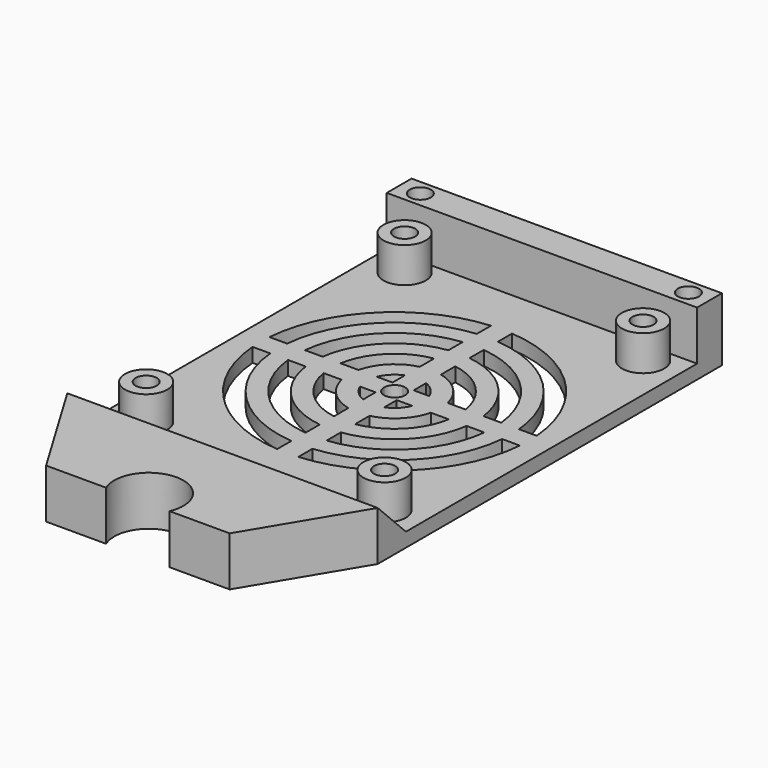
from build123d import *

# Parameters (mm, degrees)
F0_W        = 44
F0_H        = 61
F1_DEPTH    = 2
F3_DEPTH    = 7
F4_R        = 3
F4_R_2      = 1.5
F5_DEPTH    = 5
F6_T4_DEPTH = 44
F7_W        = 44
F7_H        = 4.4
F8_DEPTH    = 7
F9_R        = 1.5
F10_DEPTH   = 7
F12_DEPTH   = 2.001


# Not quite as in the source:
# - a fillet or chamfer that OpenCascade refuses, or shapes differently, is made with other operations: its cross-section is extruded or revolved along the edge and cut away or added


with BuildPart() as f1:
    # F0 (on Top) → F1 (new body)
    with BuildSketch(Plane.XY):
        Rectangle(F0_W, F0_H)
    extrude(amount=F1_DEPTH)

    # F2 (on face) → F3 (join)
    with BuildSketch(Plane(origin=(0, 0, 0), x_dir=(1, 0, 0), z_dir=(0, 0, -1))):
        with BuildLine():
            Line((-13.0117940697, 45.5), (-22, 30.5))
            Line((-22, 30.5), (22, 30.5))
            Line((22, 30.5), (13.0117940697, 45.5))
            Line((13.0117940697, 45.5), (4.5, 45.5))
            ThreePointArc((4.5, 45.5), (0, 38.660928057), (-4.5, 45.5))
            Line((-4.5, 45.5), (-13.0117940697, 45.5))
        make_face()
    extrude(amount=-F3_DEPTH)

    # F4 (on face) → F5 (join)
    with BuildSketch(Plane.XY.offset(2)):
        with Locations((-16.9, 22.9)):
            Circle(F4_R)
        with Locations((-16.9, 22.9)):
            Circle(F4_R_2, mode=Mode.SUBTRACT)
        with Locations((16.9, 22.9)):
            Circle(F4_R)
        with Locations((16.9, 22.9)):
            Circle(F4_R_2, mode=Mode.SUBTRACT)
        with Locations((16.9, -22.9)):
            Circle(F4_R)
        with Locations((16.9, -22.9)):
            Circle(F4_R_2, mode=Mode.SUBTRACT)
        with Locations((-16.9, -22.9)):
            Circle(F4_R)
        with Locations((-16.9, -22.9)):
            Circle(F4_R_2, mode=Mode.SUBTRACT)
    extrude(amount=F5_DEPTH)

    # F6: chamfer of 5 on 1 edges, made by hand


with BuildPart() as f6_tool2:
    # F6_s3 → F6_t4 (new body)
    with BuildSketch(Plane.YZ.offset(-22)):
        Polygon((-25.5, 2), (-30.5, 7), (-30.5, 2), align=None)
    extrude(amount=F6_T4_DEPTH)

    split(bisect_by=Plane(origin=(29.6352662025, -17.7578583619, 0), x_dir=(0, 0, 1), z_dir=(-0.8577903364, 0.5139997459, 0)), keep=Keep.TOP)

    split(bisect_by=Plane.XY.offset(7), keep=Keep.BOTTOM)

    split(bisect_by=Plane(origin=(-29.6352662025, -17.7578583619, 0), x_dir=(0, 0, 1), z_dir=(0.8577903364, 0.5139997459, 0)), keep=Keep.TOP)


with BuildPart() as f1_1:
    add(f1.part)

    # F6_t1: union F6_tool2
    add(f6_tool2.part)

    # F7 (on face) → F8 (join)
    with BuildSketch(Plane.XY.offset(2)):
        with Locations((0, 28.3)):
            Rectangle(F7_W, F7_H)
    extrude(amount=F8_DEPTH)

    # F9 (on face) → F10 (cut)
    with BuildSketch(Plane.XY.offset(9)):
        with Locations((-19, 28.3)):
            Circle(F9_R)
        with Locations((19, 28.3)):
            Circle(F9_R)
    extrude(amount=-F10_DEPTH, mode=Mode.SUBTRACT)

    # F11 (on face) → F12 (cut, through all)
    with BuildSketch(Plane.XY.offset(2)):
        with BuildLine():
            Line((16.4316767252, 1.5), (18.9406969249, 1.5))
            ThreePointArc((18.9406969249, 1.5), (13.4350288425, 13.4350288425), (1.5, 18.9406969249))
            Line((1.5, 18.9406969249), (1.5, 16.4316767252))
            ThreePointArc((1.5, 16.4316767252), (11.6672618896, 11.6672618896), (16.4316767252, 1.5))
        make_face()
        with BuildLine():
            ThreePointArc((1.5, -18.9406969249), (13.4350288425, -13.4350288425), (18.9406969249, -1.5))
            Line((18.9406969249, -1.5), (16.4316767252, -1.5))
            ThreePointArc((16.4316767252, -1.5), (11.6672618896, -11.6672618896), (1.5, -16.4316767252))
            Line((1.5, -16.4316767252), (1.5, -18.9406969249))
        make_face()
        with BuildLine():
            Line((-1.5, 16.4316767252), (-1.5, 18.9406969249))
            ThreePointArc((-1.5, 18.9406969249), (-13.4350288425, 13.4350288425), (-18.9406969249, 1.5))
            Line((-18.9406969249, 1.5), (-16.4316767252, 1.5))
            ThreePointArc((-16.4316767252, 1.5), (-11.6672618896, 11.6672618896), (-1.5, 16.4316767252))
        make_face()
        with BuildLine():
            Line((11.401754251, 1.5), (13.9194109071, 1.5))
            ThreePointArc((13.9194109071, 1.5), (9.8994949366, 9.8994949366), (1.5, 13.9194109071))
            Line((1.5, 13.9194109071), (1.5, 11.401754251))
            ThreePointArc((1.5, 11.401754251), (8.1317279836, 8.1317279836), (11.401754251, 1.5))
        make_face()
        with BuildLine():
            ThreePointArc((-18.9406969249, -1.5), (-13.4350288425, -13.4350288425), (-1.5, -18.9406969249))
            Line((-1.5, -18.9406969249), (-1.5, -16.4316767252))
            ThreePointArc((-1.5, -16.4316767252), (-11.6672618896, -11.6672618896), (-16.4316767252, -1.5))
            Line((-16.4316767252, -1.5), (-18.9406969249, -1.5))
        make_face()
        with BuildLine():
            ThreePointArc((1.5, -13.9194109071), (9.8994949366, -9.8994949366), (13.9194109071, -1.5))
            Line((13.9194109071, -1.5), (11.401754251, -1.5))
            ThreePointArc((11.401754251, -1.5), (8.1317279836, -8.1317279836), (1.5, -11.401754251))
            Line((1.5, -11.401754251), (1.5, -13.9194109071))
        make_face()
        with BuildLine():
            Line((-1.5, 11.401754251), (-1.5, 13.9194109071))
            ThreePointArc((-1.5, 13.9194109071), (-9.8994949366, 9.8994949366), (-13.9194109071, 1.5))
            Line((-13.9194109071, 1.5), (-11.401754251, 1.5))
            ThreePointArc((-11.401754251, 1.5), (-8.1317279836, 8.1317279836), (-1.5, 11.401754251))
        make_face()
        with BuildLine():
            Line((6.3245553203, 1.5), (8.8741196746, 1.5))
            ThreePointArc((8.8741196746, 1.5), (6.3639610307, 6.3639610307), (1.5, 8.8741196746))
            Line((1.5, 8.8741196746), (1.5, 6.3245553203))
            ThreePointArc((1.5, 6.3245553203), (4.5961940777, 4.5961940777), (6.3245553203, 1.5))
        make_face()
        with BuildLine():
            ThreePointArc((-13.9194109071, -1.5), (-9.8994949366, -9.8994949366), (-1.5, -13.9194109071))
            Line((-1.5, -13.9194109071), (-1.5, -11.401754251))
            ThreePointArc((-1.5, -11.401754251), (-8.1317279836, -8.1317279836), (-11.401754251, -1.5))
            Line((-11.401754251, -1.5), (-13.9194109071, -1.5))
        make_face()
        with BuildLine():
            ThreePointArc((1.5, -8.8741196746), (6.3639610307, -6.3639610307), (8.8741196746, -1.5))
            Line((8.8741196746, -1.5), (6.3245553203, -1.5))
            ThreePointArc((6.3245553203, -1.5), (4.5961940777, -4.5961940777), (1.5, -6.3245553203))
            Line((1.5, -6.3245553203), (1.5, -8.8741196746))
        make_face()
        with BuildLine():
            Line((-1.5, 6.3245553203), (-1.5, 8.8741196746))
            ThreePointArc((-1.5, 8.8741196746), (-6.3639610307, 6.3639610307), (-8.8741196746, 1.5))
            Line((-8.8741196746, 1.5), (-6.3245553203, 1.5))
            ThreePointArc((-6.3245553203, 1.5), (-4.5961940777, 4.5961940777), (-1.5, 6.3245553203))
        make_face()
        with BuildLine():
            Line((1.5, 1.5), (3.7080992435, 1.5))
            ThreePointArc((3.7080992435, 1.5), (2.8284271247, 2.8284271247), (1.5, 3.7080992435))
            Line((1.5, 3.7080992435), (1.5, 1.5))
        make_face()
        with BuildLine():
            ThreePointArc((-8.8741196746, -1.5), (-6.3639610307, -6.3639610307), (-1.5, -8.8741196746))
            Line((-1.5, -8.8741196746), (-1.5, -6.3245553203))
            ThreePointArc((-1.5, -6.3245553203), (-4.5961940777, -4.5961940777), (-6.3245553203, -1.5))
            Line((-6.3245553203, -1.5), (-8.8741196746, -1.5))
        make_face()
        with BuildLine():
            ThreePointArc((1.5, -3.7080992435), (2.8284271247, -2.8284271247), (3.7080992435, -1.5))
            Line((3.7080992435, -1.5), (1.5, -1.5))
            Line((1.5, -1.5), (1.5, -3.7080992435))
        make_face()
        with BuildLine():
            Line((-1.5, 1.5), (-1.5, 3.7080992435))
            ThreePointArc((-1.5, 3.7080992435), (-2.8284271247, 2.8284271247), (-3.7080992435, 1.5))
            Line((-3.7080992435, 1.5), (-1.5, 1.5))
        make_face()
        with BuildLine():
            ThreePointArc((-1.03e-08, -1.5), (1.0606601681, -1.0606601754), (1.5, 0))
            ThreePointArc((1.5, 0), (1.0606601718, 1.0606601718), (0, 1.5))
            ThreePointArc((0, 1.5), (-1.0606601711, 1.0606601725), (-1.5, 2e-09))
            ThreePointArc((-1.5, 2e-09), (-1.0606601761, -1.0606601674), (-1.03e-08, -1.5))
        make_face()
        with BuildLine():
            ThreePointArc((-3.7080992435, -1.5), (-2.8284271247, -2.8284271247), (-1.5, -3.7080992435))
            Line((-1.5, -3.7080992435), (-1.5, -1.5))
            Line((-1.5, -1.5), (-3.7080992435, -1.5))
        make_face()
    extrude(amount=-F12_DEPTH, mode=Mode.SUBTRACT)


solid = f1_1.part
